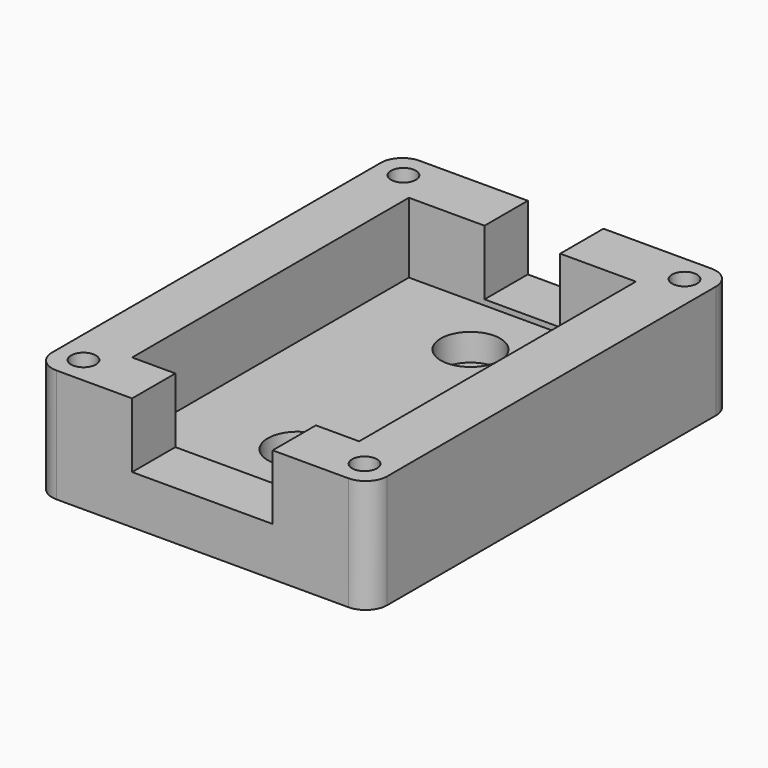
from build123d import *

# Parameters (mm, degrees)
F0_W           = 31
F0_H           = 42
F0_R           = 1.15
F0_W_2         = 21
F0_H_2         = 32
F1_DEPTH       = 6.5
F2_W           = 31
F2_H           = 42
F2_R           = 1.15
F2_W_2         = 21
F2_H_2         = 32
F3_DEPTH       = 4
F4_W           = 13
F4_H           = 5
F4_W_2         = 7
F5_DEPTH       = 6
F6_R           = 2
F8_D           = 2.9
F8_CBORE_D     = 5.5
F8_CBORE_DEPTH = 2.5


with BuildPart() as f1:
    # F0 (on Top) → F1 (new body)
    with BuildSketch(Plane.XY):
        Rectangle(F0_W, F0_H)
        with Locations((-13, -18.5)):
            Circle(F0_R, mode=Mode.SUBTRACT)
        with Locations((13, -18.5)):
            Circle(F0_R, mode=Mode.SUBTRACT)
        with Locations((-13, 18.5)):
            Circle(F0_R, mode=Mode.SUBTRACT)
        Rectangle(F0_W_2, F0_H_2, mode=Mode.SUBTRACT)
        with Locations((13, 18.5)):
            Circle(F0_R, mode=Mode.SUBTRACT)
    extrude(amount=F1_DEPTH)

    # F2 (on face) → F3 (join)
    with BuildSketch(Plane(origin=(0, 0, 0), x_dir=(1, 0, 0), z_dir=(0, 0, -1))):
        Rectangle(F2_W, F2_H)
        with Locations((-13, -18.5)):
            Circle(F2_R, mode=Mode.SUBTRACT)
        with Locations((13, -18.5)):
            Circle(F2_R, mode=Mode.SUBTRACT)
        with Locations((-13, 18.5)):
            Circle(F2_R, mode=Mode.SUBTRACT)
        Rectangle(F2_W_2, F2_H_2, mode=Mode.SUBTRACT)
        with Locations((13, 18.5)):
            Circle(F2_R, mode=Mode.SUBTRACT)
        with Locations((-13, 18.5)):
            Circle(F2_R)
        with Locations((13, 18.5)):
            Circle(F2_R)
        with Locations((-13, -18.5)):
            Circle(F2_R)
        Rectangle(F2_W_2, F2_H_2)
        with Locations((13, -18.5)):
            Circle(F2_R)
    extrude(amount=F3_DEPTH)

    # F4 (on face) → F5 (cut)
    with BuildSketch(Plane.XY.offset(6.5)):
        with Locations((0, -18.5)):
            Rectangle(F4_W, F4_H)
        with Locations((0, 18.5)):
            Rectangle(F4_W_2, F4_H)
    extrude(amount=-F5_DEPTH, mode=Mode.SUBTRACT)

    # F6
    f6_edges = [f1.edges().sort_by_distance(p)[0] for p in [
        (-15.5, 21, 1.25),
        (15.5, 21, 1.25),
        (15.5, -21, 1.25),
        (-15.5, -21, 1.25),
    ]]
    fillet(f6_edges, radius=F6_R)

    # F8 (through all)
    with Locations(Plane.XY):
        with Locations((0, 10), (0, -10)):
            CounterBoreHole(F8_D / 2, F8_CBORE_D / 2, F8_CBORE_DEPTH)


solid = f1.part
